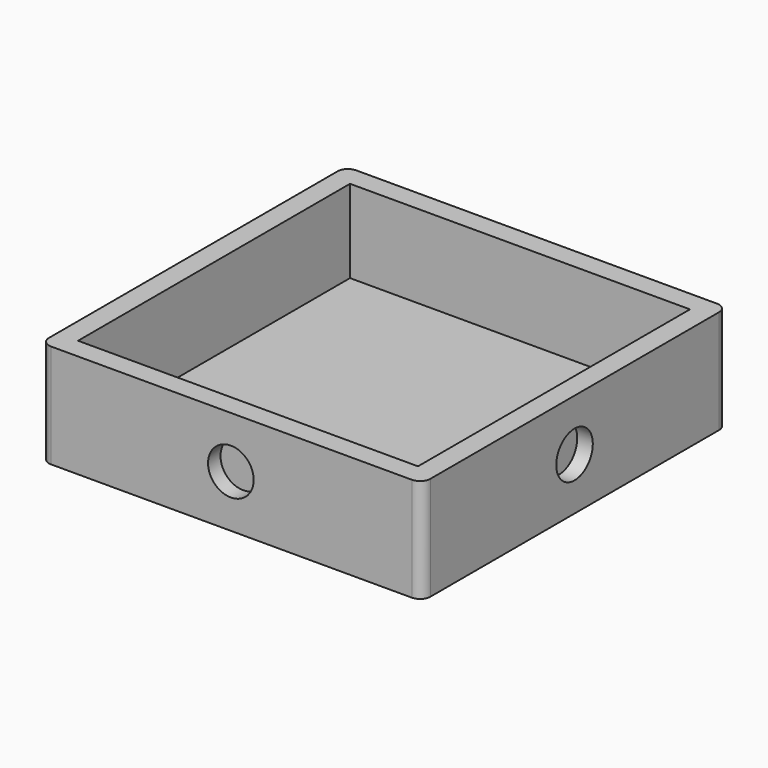
from build123d import *

# Parameters (mm, degrees)
F0_W        = 65.5
F0_H        = 65.5
F1_DEPTH    = 16
F2_T        = 4
F3_T1_DEPTH = 30
F4_R        = 4.4
F8_DEPTH    = 3
F9_DEPTH    = 3
F5_R        = 4.4
F10_DEPTH   = 3
F6_R        = 4.4
F11_DEPTH   = 3
F7_R        = 4.4
F12_DEPTH   = 3
F14_DEPTH   = 3


# Not quite as in the source:
# - a fillet or chamfer that OpenCascade refuses, or shapes differently, is made with other operations: its cross-section is extruded or revolved along the edge and cut away or added


with BuildPart() as f1:
    # F0 (on Top) → F1 (new body)
    with BuildSketch(Plane.XY):
        with Locations((4.3041806072, -3.8802318871)):
            Rectangle(F0_W, F0_H)
    extrude(amount=F1_DEPTH)

    # F2
    f2_openings = [f1.faces().sort_by_distance(p)[0] for p in [
        (4.304181, -3.880232, 16),
    ]]
    offset(amount=F2_T, openings=f2_openings, kind=Kind.INTERSECTION)

    # F3: fillet of radius 2 on 4 edges, made by hand

    # F3_s2 → F3_t1 (cut)
    with BuildSketch(Plane.XY.offset(-9)):
        with BuildLine():
            ThreePointArc((41.0541806072, -38.6302318871), (40.4683941696, -40.0444454495), (39.0541806072, -40.6302318871))
            Line((39.0541806072, -40.6302318871), (41.0541806072, -40.6302318871))
            Line((41.0541806072, -40.6302318871), (41.0541806072, -38.6302318871))
        make_face()
        with BuildLine():
            ThreePointArc((41.0541806072, 30.8697681129), (40.4683941696, 32.2839816753), (39.0541806072, 32.8697681129))
            Line((39.0541806072, 32.8697681129), (41.0541806072, 32.8697681129))
            Line((41.0541806072, 32.8697681129), (41.0541806072, 30.8697681129))
        make_face()
        with BuildLine():
            ThreePointArc((-30.4458193928, 32.8697681129), (-31.8600329552, 32.2839816753), (-32.4458193928, 30.8697681129))
            Line((-32.4458193928, 30.8697681129), (-32.4458193928, 32.8697681129))
            Line((-32.4458193928, 32.8697681129), (-30.4458193928, 32.8697681129))
        make_face()
        with BuildLine():
            ThreePointArc((-32.4458193928, -38.6302318871), (-31.8600329552, -40.0444454495), (-30.4458193928, -40.6302318871))
            Line((-30.4458193928, -40.6302318871), (-32.4458193928, -40.6302318871))
            Line((-32.4458193928, -40.6302318871), (-32.4458193928, -38.6302318871))
        make_face()
    extrude(amount=F3_T1_DEPTH, mode=Mode.SUBTRACT)

    # F4 (on face) → F8 (join)
    with BuildSketch(Plane(origin=(-32.4458193928, 0, 0), x_dir=(0, -1, 0), z_dir=(-1, 0, 0))):
        with Locations((3.8802318871, 6)):
            Circle(F4_R)
    extrude(amount=-F8_DEPTH)

    # F4 (on face) → F9 (cut)
    with BuildSketch(Plane(origin=(-32.4458193928, 0, 0), x_dir=(0, -1, 0), z_dir=(-1, 0, 0))):
        with Locations((3.8802318871, 6)):
            Circle(F4_R)
    extrude(amount=-F9_DEPTH, mode=Mode.SUBTRACT)

    # F5 (on face) → F10 (cut)
    with BuildSketch(Plane.XZ.offset(40.6302318871)):
        with Locations((4.2000180173, 6.0547004089)):
            Circle(F5_R)
    extrude(amount=-F10_DEPTH, mode=Mode.SUBTRACT)

    # F6 (on face) → F11 (cut)
    with BuildSketch(Plane.YZ.offset(41.0541806072)):
        with Locations((-3.9293510383, 6.0207889489)):
            Circle(F6_R)
    extrude(amount=-F11_DEPTH, mode=Mode.SUBTRACT)

    # F7 (on face) → F12 (cut)
    with BuildSketch(Plane(origin=(0, 32.8697681129, 0), x_dir=(-1, 0, 0), z_dir=(0, 1, 0))):
        with Locations((-4.345219037, 6.0662772571)):
            Circle(F7_R)
    extrude(amount=-F12_DEPTH, mode=Mode.SUBTRACT)

    # F13 (on face) → F14 (cut)
    with BuildSketch(Plane(origin=(0, 0, -4), x_dir=(1, 0, 0), z_dir=(0, 0, -1))):
        Polygon((27.9313208005, 18.9403499991), (20.8531849213, 26.0043426715), (-15.9149708404, -10.7666407574), (-8.8368349613, -17.8306334298), align=None)
    extrude(amount=-F14_DEPTH, mode=Mode.SUBTRACT)


solid = f1.part
